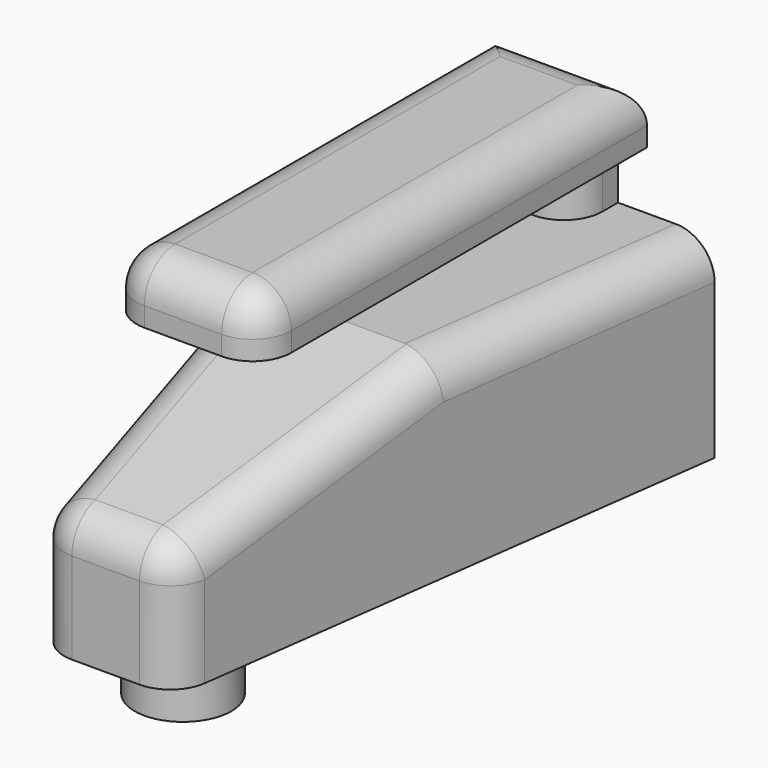
from build123d import *

# Parameters (mm, degrees)
F0_W      = 1.5
F0_H      = 1
F1_DEPTH  = 3
F3_DEPTH  = 25
F5_DEPTH  = 25
F6_R      = 0.25
F7_DEPTH  = 0.3
F8_W      = 0.5
F8_H      = 0.3
F9_DEPTH  = 0.3
F10_W     = 0.5
F10_H     = 0.3
F11_DEPTH = 0.3
F12_R     = 0.2
F13_R     = 0.2


with BuildPart() as f1:
    # F0 (on Front) → F1 (new body)
    with BuildSketch(Plane.XZ):
        with Locations((0.75, 0.5)):
            Rectangle(F0_W, F0_H)
    extrude(amount=F1_DEPTH)

    # F2 (on face) → F3 (cut)
    with BuildSketch(Plane.YZ.offset(1.5)):
        Polygon((-3, 1), (-3, 0.6286599091), (-1.5, 1), align=None)
    extrude(amount=-F3_DEPTH, mode=Mode.SUBTRACT)

    # F4 (on face) → F5 (cut)
    with BuildSketch(Plane.XY.offset(1)):
        Polygon((1.5, -1.5), (1.5, 0), (1.3, -1.5), align=None)
        Polygon((1.5, -1.5), (1.3, -1.5), (1.1, -3), (1.5, -3), align=None)
        Polygon((0.2, -1.5), (0, 0), (0, -1.5), align=None)
        Polygon((0.4, -3), (0.2, -1.5), (0, -1.5), (0, -3), align=None)
    extrude(amount=-F5_DEPTH, mode=Mode.SUBTRACT)

    # F6 (on face) → F7 (join)
    with BuildSketch(Plane(origin=(0, 0, 0), x_dir=(1, 0, 0), z_dir=(0, 0, -1))):
        with Locations((0.75, 2.5)):
            Circle(F6_R)
    extrude(amount=F7_DEPTH)

    # F8 (on face) → F9 (join)
    with BuildSketch(Plane.XY.offset(1)):
        with Locations((0.75, -0.15)):
            Rectangle(F8_W, F8_H)
    extrude(amount=F9_DEPTH)

    # F10 (on face) → F11 (join)
    with BuildSketch(Plane.XY.offset(1.3)):
        Polygon((0.5, 0), (0.35, 0), (0.35, -2.5), (1.15, -2.5), (1.15, 0), (1, 0), (1, -0.3), (0.5, -0.3), align=None)
        with Locations((0.75, -0.15)):
            Rectangle(F10_W, F10_H)
    extrude(amount=F11_DEPTH)

    # F12
    f12_edges = [f1.edges().sort_by_distance(p)[0] for p in [
        (1.2, -2.25, 0.81433),
        (0.3, -2.25, 0.81433),
        (0.75, -3, 0.62866),
        (1.4, -0.75, 1),
        (0.1, -0.75, 1),
        (0.4, -3, 0.31433),
        (1.1, -3, 0.31433),
    ]]
    fillet(f12_edges, radius=F12_R)

    # F13
    f13_edges = [f1.edges().sort_by_distance(p)[0] for p in [
        (1, -0.3, 1.15),
        (0.5, -0.3, 1.15),
        (0.35, -2.5, 1.45),
        (1.15, -2.5, 1.45),
        (0.75, -2.5, 1.6),
        (0.35, -1.25, 1.6),
        (1.15, -1.25, 1.6),
        (0.75, 0, 1.6),
    ]]
    fillet(f13_edges, radius=F13_R)


solid = f1.part
